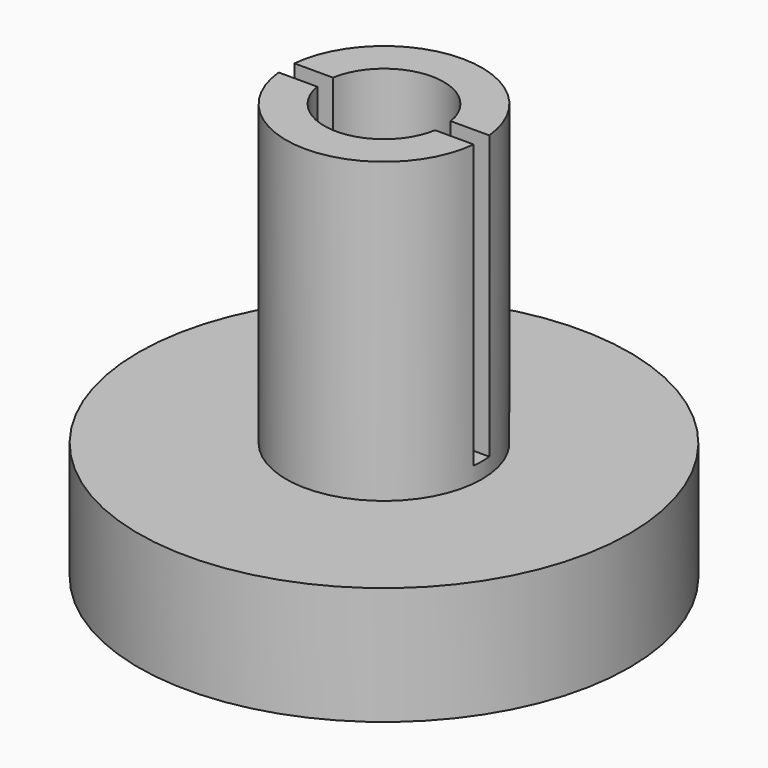
from build123d import *

# Parameters (mm, degrees)
F0_R     = 39.6875
F0_R_2   = 9.652
F1_DEPTH = 19.05
F2_R     = 15.8369
F2_R_2   = 9.652
F3_DEPTH = 48.26
F4_R     = 2.4645418127
F5_DEPTH = 12.7
F7_DEPTH = 45.72


with BuildPart() as f1:
    # F0 (on Top) → F1 (new body)
    with BuildSketch(Plane.XY):
        Circle(F0_R)
        Circle(F0_R_2, mode=Mode.SUBTRACT)
    extrude(amount=F1_DEPTH)

    # F2 (on face) → F3 (join)
    with BuildSketch(Plane.XY.offset(19.05)):
        Circle(F2_R)
        Circle(F2_R_2, mode=Mode.SUBTRACT)
    extrude(amount=F3_DEPTH)

    # F4 (on face) → F5 (cut)
    with BuildSketch(Plane(origin=(0, 0, 0), x_dir=(1, 0, 0), z_dir=(0, 0, -1))):
        with Locations((-31.75, 0)):
            Circle(F4_R)
        with Locations((0, -31.75)):
            Circle(F4_R)
        with Locations((0, 31.75)):
            Circle(F4_R)
        with Locations((31.75, 0)):
            Circle(F4_R)
    extrude(amount=-F5_DEPTH, mode=Mode.SUBTRACT)

    # F6 (on face) → F7 (cut)
    with BuildSketch(Plane.XY.offset(67.31)):
        with BuildLine():
            Line((15.757133158, -1.5875), (25.4, -1.5875))
            Line((25.4, -1.5875), (25.4, 1.5875))
            Line((25.4, 1.5875), (15.757133158, 1.5875))
            ThreePointArc((15.757133158, 1.5875), (15.8169457184, 0.7947513761), (15.8369, 0))
            ThreePointArc((15.8369, 0), (15.8169457184, -0.7947513761), (15.757133158, -1.5875))
        make_face()
        with BuildLine():
            Line((9.5205539623, -1.5875), (15.757133158, -1.5875))
            ThreePointArc((15.757133158, -1.5875), (15.8169457184, -0.7947513761), (15.8369, 0))
            ThreePointArc((15.8369, 0), (15.8169457184, 0.7947513761), (15.757133158, 1.5875))
            Line((15.757133158, 1.5875), (9.5205539623, 1.5875))
            ThreePointArc((9.5205539623, 1.5875), (9.6190823586, 0.7964663067), (9.652, 0))
            ThreePointArc((9.652, 0), (9.6190823586, -0.7964663067), (9.5205539623, -1.5875))
        make_face()
        with BuildLine():
            ThreePointArc((-15.757133158, 1.5875), (-15.8369, 0), (-15.757133158, -1.5875))
            Line((-15.757133158, -1.5875), (-9.5205539623, -1.5875))
            ThreePointArc((-9.5205539623, -1.5875), (-9.652, 0), (-9.5205539623, 1.5875))
            Line((-9.5205539623, 1.5875), (-15.757133158, 1.5875))
        make_face()
        with BuildLine():
            Line((-25.4, -1.5875), (-15.757133158, -1.5875))
            ThreePointArc((-15.757133158, -1.5875), (-15.8369, 0), (-15.757133158, 1.5875))
            Line((-15.757133158, 1.5875), (-25.4, 1.5875))
            Line((-25.4, 1.5875), (-25.4, -1.5875))
        make_face()
    extrude(amount=-F7_DEPTH, mode=Mode.SUBTRACT)


solid = f1.part
